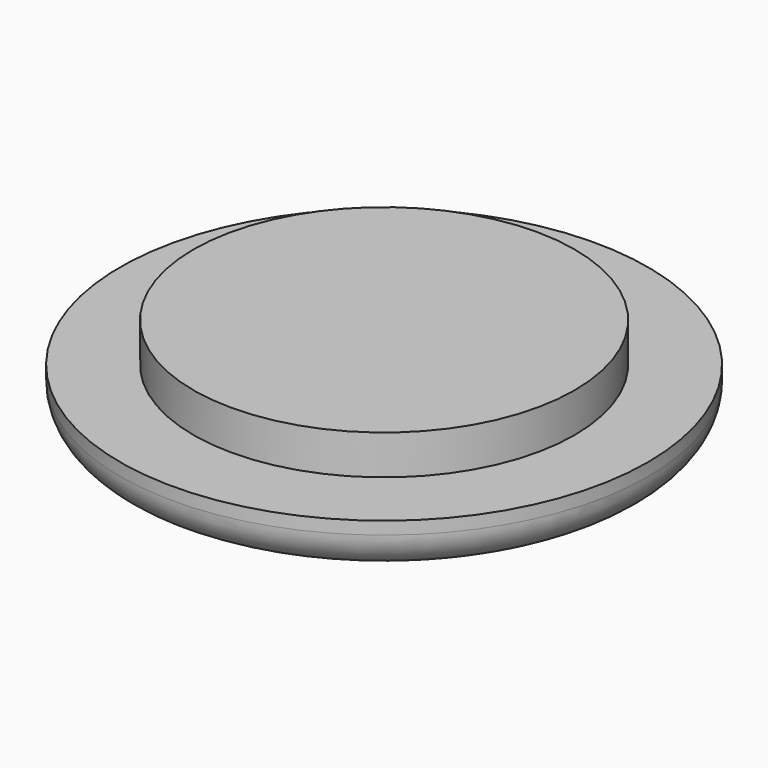
from build123d import *

# Parameters (mm, degrees)
F0_R     = 35.4529924148
F0_R_2   = 26.5998947574
F1_DEPTH = 12
F2_R     = 20.3647706408
F3_DEPTH = 4
F5_R     = 5
F6_R     = 5
F7_R     = 35.4529924148
F7_R_2   = 25.6021329211
F8_DEPTH = 5.3


# Not quite as in the source:
# - a fillet or chamfer that OpenCascade refuses, or shapes differently, is made with other operations: its cross-section is extruded or revolved along the edge and cut away or added


with BuildPart() as f1:
    # F0 (on Top) → F1 (new body)
    with BuildSketch(Plane.XY):
        Circle(F0_R)
        Circle(F0_R_2, mode=Mode.SUBTRACT)
        Circle(F0_R_2)
    extrude(amount=F1_DEPTH)

    # F2 (on face) → F3 (cut)
    with BuildSketch(Plane(origin=(0, 0, 0), x_dir=(1, 0, 0), z_dir=(0, 0, -1))):
        Circle(F2_R)
    extrude(amount=-F3_DEPTH, mode=Mode.SUBTRACT)

    # F4: fillet of radius 5 on 1 edges, made by hand

    # F4_s1 → F4_t2 (revolve)
    with BuildSketch(Plane.XZ):
        with BuildLine():
            ThreePointArc((20.3647706408, 0), (18.6280688154, 2.8729833462), (15.4657911552, 4))
            Line((15.4657911552, 4), (20.3647706408, 4))
            Line((20.3647706408, 4), (20.3647706408, 0))
        make_face()
    revolve(axis=Axis((0, 0, 4), (0, 0, -1)))

    # F5
    f5_edges = [f1.edges().sort_by_distance(p)[0] for p in [
        (-20.364771, 0, 0),
    ]]
    fillet(f5_edges, radius=F5_R)

    # F6
    f6_edges = [f1.edges().sort_by_distance(p)[0] for p in [
        (-35.452992, 0, 0),
    ]]
    fillet(f6_edges, radius=F6_R)

    # F7 (on face) → F8 (cut)
    with BuildSketch(Plane.XY.offset(12)):
        Circle(F7_R)
        Circle(F7_R_2, mode=Mode.SUBTRACT)
    extrude(amount=-F8_DEPTH, mode=Mode.SUBTRACT)


solid = f1.part
